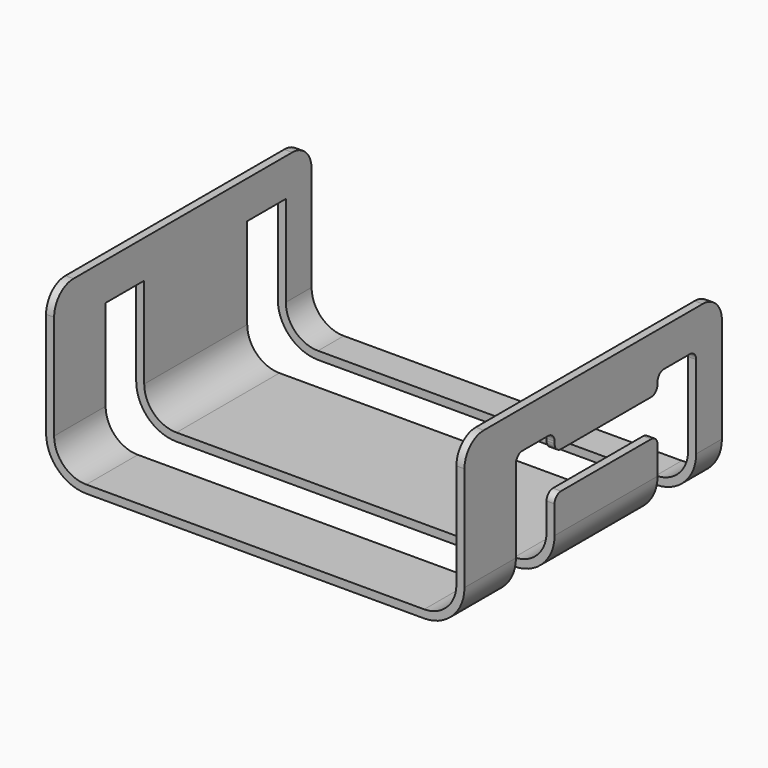
from build123d import *

# Parameters (mm, degrees)
F2_DEPTH = 200
F3_W     = 30
F3_H     = 100
F4_DEPTH = 500
F6_R     = 15
F7_R     = 5
F8_W     = 101.1056527495
F8_H     = 22.9697218165
F9_DEPTH = 200
F10_R    = 5


with BuildPart() as f2:
    # F0 (on Front) → F2 (new body)
    with BuildSketch(Plane.XZ):
        with BuildLine():
            Line((-127.5536519289, -36.5021181107), (-127.5536519289, 43.4978818893))
            Line((-127.5536519289, 43.4978818893), (-132.5536519289, 43.4978818893))
            Line((-132.5536519289, 43.4978818893), (-132.5536519289, -36.5021181107))
            ThreePointArc((-132.5536519289, -36.5021181107), (-125.2313214586, -54.1797876403), (-107.5536519289, -61.5021181107))
            Line((-107.5536519289, -61.5021181107), (102.4463480711, -61.5021181107))
            ThreePointArc((102.4463480711, -61.5021181107), (120.1240176008, -54.1797876403), (127.4463480711, -36.5021181107))
            Line((127.4463480711, -36.5021181107), (127.4463480711, 43.4978818893))
            Line((127.4463480711, 43.4978818893), (122.4463480711, 43.4978818893))
            Line((122.4463480711, 43.4978818893), (122.4463480711, -36.5021181107))
            ThreePointArc((122.4463480711, -36.5021181107), (116.5884836948, -50.6442537344), (102.4463480711, -56.5021181107))
            Line((102.4463480711, -56.5021181107), (-107.5536519289, -56.5021181107))
            ThreePointArc((-107.5536519289, -56.5021181107), (-121.6957875526, -50.6442537344), (-127.5536519289, -36.5021181107))
        make_face()
    extrude(amount=F2_DEPTH)


with BuildPart() as f4:
    # F3 (on offset) → F4 (new body)
    with BuildSketch(Plane.YZ.offset(200)):
        with Locations((-145, -29.9103426556)):
            Rectangle(F3_W, F3_H)
    extrude(amount=-F4_DEPTH)


with BuildPart() as f4b:
    # F3 (on offset) → F4, piece 2 (new body)
    with BuildSketch(Plane.YZ.offset(200)):
        with Locations((-35, -29.9103426556)):
            Rectangle(F3_W, F3_H)
    extrude(amount=-F4_DEPTH)


with BuildPart() as f2_1:
    add(f2.part)

    # F5: cut F4, F4b
    add(f4.part, mode=Mode.SUBTRACT)
    add(f4b.part, mode=Mode.SUBTRACT)

    # F6
    f6_edges = [f2_1.edges().sort_by_distance(p)[0] for p in [
        (-130.053652, -200, 43.497882),
        (-130.053652, 0, 43.497882),
        (124.946348, -200, 43.497882),
        (124.946348, 0, 43.497882),
    ]]
    fillet(f6_edges, radius=F6_R)

    # F7
    f7_edges = [f2_1.edges().sort_by_distance(p)[0] for p in [
        (124.946348, -20, 20.089657),
        (124.946348, -50, 20.089657),
    ]]
    fillet(f7_edges, radius=F7_R)

    # F8 (on offset) → F9 (cut)
    with BuildSketch(Plane.YZ.offset(200)):
        with Locations((-91.6927345097, -2.6946733706)):
            Rectangle(F8_W, F8_H)
    extrude(amount=-F9_DEPTH, mode=Mode.SUBTRACT)

    # F10
    f10_edges = [f2_1.edges().sort_by_distance(p)[0] for p in [
        (124.946348, -50, -14.179534),
        (124.946348, -50, 8.790188),
        (124.946348, -130, 8.790188),
        (124.946348, -130, -14.179534),
        (124.946348, -130, 20.089657),
        (124.946348, -160, 20.089657),
    ]]
    fillet(f10_edges, radius=F10_R)


solid = f2_1.part
